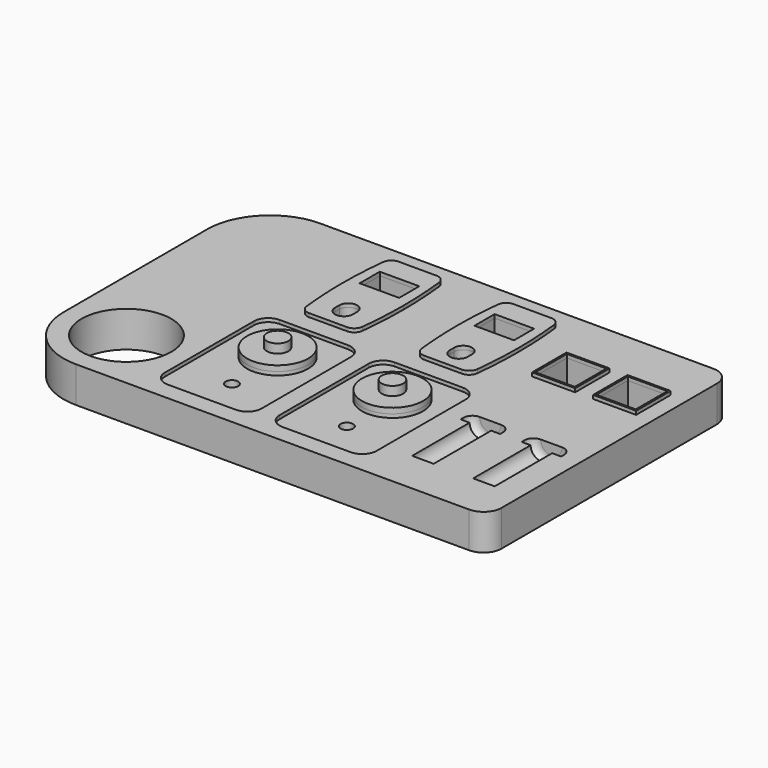
from build123d import *

# Parameters (mm, degrees)
F0_R          = 12.5
F1_DEPTH      = 10
F2_R          = 1.75
F2_R_2        = 8.5
F3_DEPTH      = 1
F4_DEPTH      = 7
F2_R_3        = 3
F5_DEPTH      = 1.5
F6_DEPTH      = 4
F2_W          = 11
F2_H          = 7
F7_DEPTH      = 1
F8_DEPTH      = 9
F9_DEPTH      = 6
F2_W_2        = 12
F2_H_2        = 12
F2_H_3        = 11
F12_DEPTH     = 1
F13_DEPTH     = 8
F14_TEXT_SIZE = 5.5555555556
F15_DEPTH     = 1


# Not quite as in the source:
# - Text() gives the source's letters only with a copy of the font that has no kerning and outlines rounded to 1/6400 em; it was checked with that copy


with BuildPart() as f1:
    # F0 (on Top) → F1 (new body)
    with BuildSketch(Plane.XY):
        with BuildLine():
            ThreePointArc((0, 17.5), (5.1256313292, 5.1256313292), (17.5, 0))
            Line((17.5, 0), (127, 0))
            ThreePointArc((127, 0), (130.5355339059, 1.4644660941), (132, 5))
            Line((132, 5), (132, 80))
            ThreePointArc((132, 80), (130.5355339059, 83.5355339059), (127, 85))
            Line((127, 85), (17.5, 85))
            ThreePointArc((17.5, 85), (5.1256313292, 79.8743686708), (0, 67.5))
            Line((0, 67.5), (0, 17.5))
        make_face()
        with Locations((17.5, 17.5)):
            Circle(F0_R, mode=Mode.SUBTRACT)
    extrude(amount=F1_DEPTH)

    # F2 (on face) → F3 (cut)
    with BuildSketch(Plane.XY.offset(10)):
        with BuildLine():
            ThreePointArc((35, 9), (36.1715728753, 6.1715728753), (39, 5))
            Line((39, 5), (58, 5))
            ThreePointArc((58, 5), (60.8284271247, 6.1715728753), (62, 9))
            Line((62, 9), (62, 40))
            ThreePointArc((62, 40), (60.8284271247, 42.8284271247), (58, 44))
            Line((58, 44), (39, 44))
            ThreePointArc((39, 44), (36.1715728753, 42.8284271247), (35, 40))
            Line((35, 40), (35, 9))
        make_face()
        with Locations((48.5, 15.5)):
            Circle(F2_R, mode=Mode.SUBTRACT)
        with Locations((48.5, 31.4)):
            Circle(F2_R_2, mode=Mode.SUBTRACT)
        with BuildLine():
            ThreePointArc((67, 9), (68.1715728753, 6.1715728753), (71, 5))
            Line((71, 5), (90, 5))
            ThreePointArc((90, 5), (92.8284271247, 6.1715728753), (94, 9))
            Line((94, 9), (94, 40))
            ThreePointArc((94, 40), (92.8284271247, 42.8284271247), (90, 44))
            Line((90, 44), (71, 44))
            ThreePointArc((71, 44), (68.1715728753, 42.8284271247), (67, 40))
            Line((67, 40), (67, 9))
        make_face()
        with Locations((80.5, 15.5)):
            Circle(F2_R, mode=Mode.SUBTRACT)
        with Locations((80.5, 31.4)):
            Circle(F2_R_2, mode=Mode.SUBTRACT)
    extrude(amount=-F3_DEPTH, mode=Mode.SUBTRACT)

    # F2 (on face) → F4 (cut)
    with BuildSketch(Plane.XY.offset(10)):
        with Locations((48.5, 15.5)):
            Circle(F2_R)
        with Locations((80.5, 15.5)):
            Circle(F2_R)
    extrude(amount=-F4_DEPTH, mode=Mode.SUBTRACT)

    # F2 (on face) → F5 (join)
    with BuildSketch(Plane.XY.offset(10)):
        with Locations((80.5, 31.4)):
            Circle(F2_R_2)
        with Locations((80.5, 31.4)):
            Circle(F2_R_3, mode=Mode.SUBTRACT)
        with Locations((48.5, 31.4)):
            Circle(F2_R_2)
        with Locations((48.5, 31.4)):
            Circle(F2_R_3, mode=Mode.SUBTRACT)
    extrude(amount=F5_DEPTH)

    # F2 (on face) → F6 (join)
    with BuildSketch(Plane.XY.offset(10)):
        with Locations((48.5, 31.4)):
            Circle(F2_R_3)
        with Locations((80.5, 31.4)):
            Circle(F2_R_3)
    extrude(amount=F6_DEPTH)

    # F2 (on face) → F7 (join)
    with BuildSketch(Plane.XY.offset(10)):
        with BuildLine():
            ThreePointArc((40.7334241181, 51.2256126407), (41.5503832225, 49.6377475469), (43.2183208115, 49))
            Line((43.2183208115, 49), (53.7816791885, 49))
            ThreePointArc((53.7816791885, 49), (55.4496167775, 49.6377475469), (56.2665758819, 51.2256126407))
            ThreePointArc((56.2665758819, 51.2256126407), (56.8165052968, 57.8777213518), (57, 64.55))
            ThreePointArc((57, 64.55), (56.8165052968, 71.2222786482), (56.2665758819, 77.8743873593))
            ThreePointArc((56.2665758819, 77.8743873593), (55.4496167775, 79.4622524531), (53.7816791885, 80.1))
            Line((53.7816791885, 80.1), (43.2183208115, 80.1))
            ThreePointArc((43.2183208115, 80.1), (41.5503832225, 79.4622524531), (40.7334241181, 77.8743873593))
            ThreePointArc((40.7334241181, 77.8743873593), (40.1834947032, 71.2222786482), (40, 64.55))
            ThreePointArc((40, 64.55), (40.1834947032, 57.8777213518), (40.7334241181, 51.2256126407))
        make_face()
        with BuildLine():
            Line((51, 56), (51, 54.5))
            ThreePointArc((51, 54.5), (48.5, 52), (46, 54.5))
            Line((46, 54.5), (46, 56))
            ThreePointArc((46, 56), (48.5, 58.5), (51, 56))
        make_face(mode=Mode.SUBTRACT)
        with Locations((48.5, 70.35)):
            Rectangle(F2_W, F2_H, mode=Mode.SUBTRACT)
        with BuildLine():
            ThreePointArc((72.7334241181, 51.2256126407), (73.5503832225, 49.6377475469), (75.2183208115, 49))
            Line((75.2183208115, 49), (85.7816791885, 49))
            ThreePointArc((85.7816791885, 49), (87.4496167775, 49.6377475469), (88.2665758819, 51.2256126407))
            ThreePointArc((88.2665758819, 51.2256126407), (88.8165052968, 57.8777213518), (89, 64.55))
            ThreePointArc((89, 64.55), (88.8165052968, 71.2222786482), (88.2665758819, 77.8743873593))
            ThreePointArc((88.2665758819, 77.8743873593), (87.4496167775, 79.4622524531), (85.7816791885, 80.1))
            Line((85.7816791885, 80.1), (75.2183208115, 80.1))
            ThreePointArc((75.2183208115, 80.1), (73.5503832225, 79.4622524531), (72.7334241181, 77.8743873593))
            ThreePointArc((72.7334241181, 77.8743873593), (72.1834947032, 71.2222786482), (72, 64.55))
            ThreePointArc((72, 64.55), (72.1834947032, 57.8777213518), (72.7334241181, 51.2256126407))
        make_face()
        with BuildLine():
            Line((83, 56), (83, 54.5))
            ThreePointArc((83, 54.5), (80.5, 52), (78, 54.5))
            Line((78, 54.5), (78, 56))
            ThreePointArc((78, 56), (80.5, 58.5), (83, 56))
        make_face(mode=Mode.SUBTRACT)
        with Locations((80.5, 70.35)):
            Rectangle(F2_W, F2_H, mode=Mode.SUBTRACT)
    extrude(amount=F7_DEPTH)

    # F2 (on face) → F8 (cut)
    with BuildSketch(Plane.XY.offset(10)):
        with Locations((48.5, 70.35)):
            Rectangle(F2_W, F2_H)
        with Locations((80.5, 70.35)):
            Rectangle(F2_W, F2_H)
    extrude(amount=-F8_DEPTH, mode=Mode.SUBTRACT)

    # F2 (on face) → F9 (cut)
    with BuildSketch(Plane.XY.offset(10)):
        with BuildLine():
            ThreePointArc((46, 54.5), (48.5, 52), (51, 54.5))
            Line((51, 54.5), (51, 56))
            ThreePointArc((51, 56), (48.5, 58.5), (46, 56))
            Line((46, 56), (46, 54.5))
        make_face()
        with BuildLine():
            ThreePointArc((78, 54.5), (80.5, 52), (83, 54.5))
            Line((83, 54.5), (83, 56))
            ThreePointArc((83, 56), (80.5, 58.5), (78, 56))
            Line((78, 56), (78, 54.5))
        make_face()
    extrude(amount=-F9_DEPTH, mode=Mode.SUBTRACT)

    # F2 (on face) → F10 (revolve, cut)
    with BuildSketch(Plane.XY.offset(10)):
        with BuildLine():
            Line((104.5, 32), (104.5, 12))
            Line((104.5, 12), (107.5, 12))
            Line((107.5, 12), (107.5, 32))
            Line((107.5, 32), (110, 32))
            Line((110, 32), (110, 33))
            ThreePointArc((110, 33), (109.267766953, 34.767766953), (107.5, 35.5))
            Line((107.5, 35.5), (104.5, 35.5))
            Line((104.5, 35.5), (104.5, 32))
        make_face()
    revolve(axis=Axis((104.5, 22, 10), (0, 1, 0)), mode=Mode.SUBTRACT)

    # F2 (on face) → F11 (revolve, cut)
    with BuildSketch(Plane.XY.offset(10)):
        with BuildLine():
            Line((121.5, 32), (121.5, 12))
            Line((121.5, 12), (124.5, 12))
            Line((124.5, 12), (124.5, 32))
            Line((124.5, 32), (127, 32))
            Line((127, 32), (127, 33))
            ThreePointArc((127, 33), (126.267766953, 34.767766953), (124.5, 35.5))
            Line((124.5, 35.5), (121.5, 35.5))
            Line((121.5, 35.5), (121.5, 32))
        make_face()
    revolve(axis=Axis((121.5, 22, 10), (0, 1, 0)), mode=Mode.SUBTRACT)

    # F2 (on face) → F12 (join)
    with BuildSketch(Plane.XY.offset(10)):
        with Locations((121.5, 63.5)):
            Rectangle(F2_W_2, F2_H_2)
        with Locations((121.5, 63.5)):
            Rectangle(F2_W, F2_H_3, mode=Mode.SUBTRACT)
        with Locations((104.5, 63.5)):
            Rectangle(F2_W_2, F2_H_2)
        with Locations((104.5, 63.5)):
            Rectangle(F2_W, F2_H_3, mode=Mode.SUBTRACT)
    extrude(amount=F12_DEPTH)

    # F2 (on face) → F13 (cut)
    with BuildSketch(Plane.XY.offset(10)):
        with Locations((104.5, 63.5)):
            Rectangle(F2_W, F2_H_3)
        with Locations((121.5, 63.5)):
            Rectangle(F2_W, F2_H_3)
    extrude(amount=-F13_DEPTH, mode=Mode.SUBTRACT)

    # F14 (on face) → F15 (cut)
    with BuildSketch(Plane(origin=(0, 0, 0), x_dir=(1, 0, 0), z_dir=(0, 0, -1))):
        with Locations((30, -9)):
            Text('969, 970', F14_TEXT_SIZE, font='Open Sans', text_align=(TextAlign.LEFT, TextAlign.BOTTOM))
    extrude(amount=-F15_DEPTH, mode=Mode.SUBTRACT)


solid = f1.part
